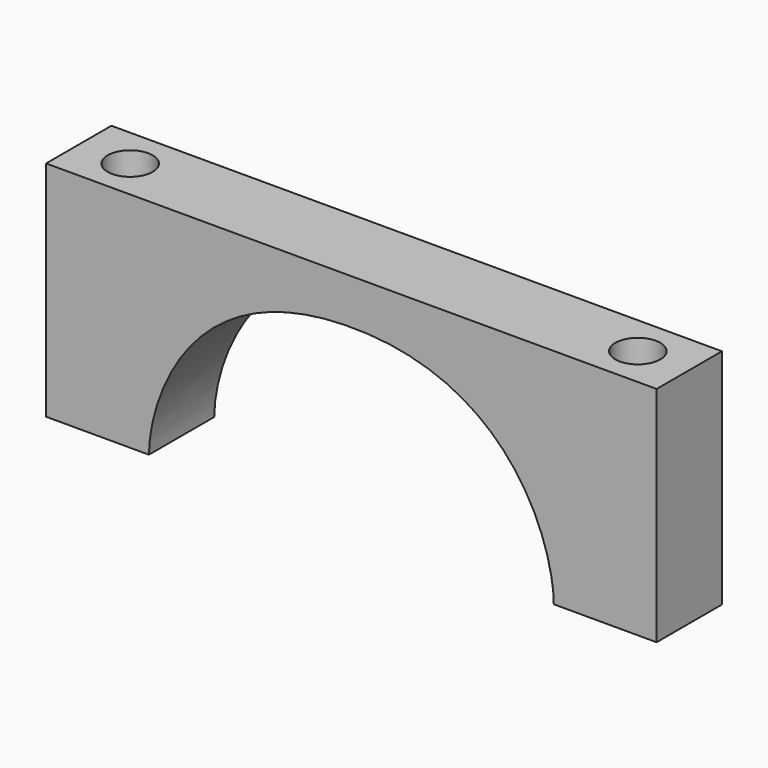
from build123d import *

# Parameters (mm, degrees)
F1_DEPTH = 12.7
F2_R     = 3.5
F3_DEPTH = 34.7010003931


with BuildPart() as f1:
    # F0 (on Front) → F1 (new body)
    with BuildSketch(Plane.XZ):
        with BuildLine():
            Line((-7.0000002931, 0), (0, 0))
            add(Edge.make_bspline(
                [(0, 0), (0, 7.4632624164), (6.0286673327, 27.7), (31.5, 27.7)],
                knots=[0, 0, 0, 0, 41.9468711586, 41.9468711586, 41.9468711586, 41.9468711586], degree=3))
            Line((31.5, 27.7), (31.5, 34.7000002931))
            Line((31.5, 34.7000002931), (27.8526304737, 34.7000002931))
            add(Edge.make_bspline(
                [(-7.0000002931, 0), (-7.0039994936, 0.2340387149), (-7.0037511705, 0.948501906), (-6.9151085802, 2.7064518501), (-6.5108229743, 5.6903444563), (-5.45581027, 10.1440145543), (-3.2381450913, 15.5278434101), (0.3694739726, 21.3486442297), (5.587224769, 26.85724492), (12.594863214, 31.3943142529), (20.2705683515, 34.1506367566), (25.5784159374, 34.6301697858), (27.8526304737, 34.7000002931)],
                knots=[0, 0, 0, 0, 0.7020561458, 2.1432682107, 5.2767521047, 9.7221639973, 15.8389070563, 22.6581648152, 30.1626757657, 38.4005606449, 47.497203749, 54.3101388825, 54.3101388825, 54.3101388825, 54.3101388825], degree=3))
        make_face()
        with BuildLine():
            Line((31.5, 34.7000002931), (31.5, 27.7))
            add(Edge.make_bspline(
                [(63, 0), (63, 7.4632624164), (56.9713326673, 27.7), (31.5, 27.7)],
                knots=[0, 0, 0, 0, 41.9468711586, 41.9468711586, 41.9468711586, 41.9468711586], degree=3))
            Line((63, 0), (79, 0))
            Line((79, 0), (79, 34.7000002931))
            Line((79, 34.7000002931), (31.5, 34.7000002931))
        make_face()
        with BuildLine():
            Line((-16, 0), (-7.0000002931, 0))
            add(Edge.make_bspline(
                [(-7.0000002931, 0), (-7.0039994936, 0.2340387149), (-7.0037511705, 0.948501906), (-6.9151085802, 2.7064518501), (-6.5108229743, 5.6903444563), (-5.45581027, 10.1440145543), (-3.2381450913, 15.5278434101), (0.3694739726, 21.3486442297), (5.587224769, 26.85724492), (12.594863214, 31.3943142529), (20.2705683515, 34.1506367566), (25.5784159374, 34.6301697858), (27.8526304737, 34.7000002931)],
                knots=[0, 0, 0, 0, 0.7020561458, 2.1432682107, 5.2767521047, 9.7221639973, 15.8389070563, 22.6581648152, 30.1626757657, 38.4005606449, 47.497203749, 54.3101388825, 54.3101388825, 54.3101388825, 54.3101388825], degree=3))
            Line((27.8526304737, 34.7000002931), (-16, 34.7000002931))
            Line((-16, 34.7000002931), (-16, 0))
        make_face()
    extrude(amount=F1_DEPTH)

    # F2 (on face) → F3 (cut, through all)
    with BuildSketch(Plane(origin=(0, 0, 0), x_dir=(1, 0, 0), z_dir=(0, 0, -1))):
        with Locations((-8, 6.35)):
            Circle(F2_R)
        with Locations((71, 6.35)):
            Circle(F2_R)
    extrude(amount=-F3_DEPTH, mode=Mode.SUBTRACT)


solid = f1.part
